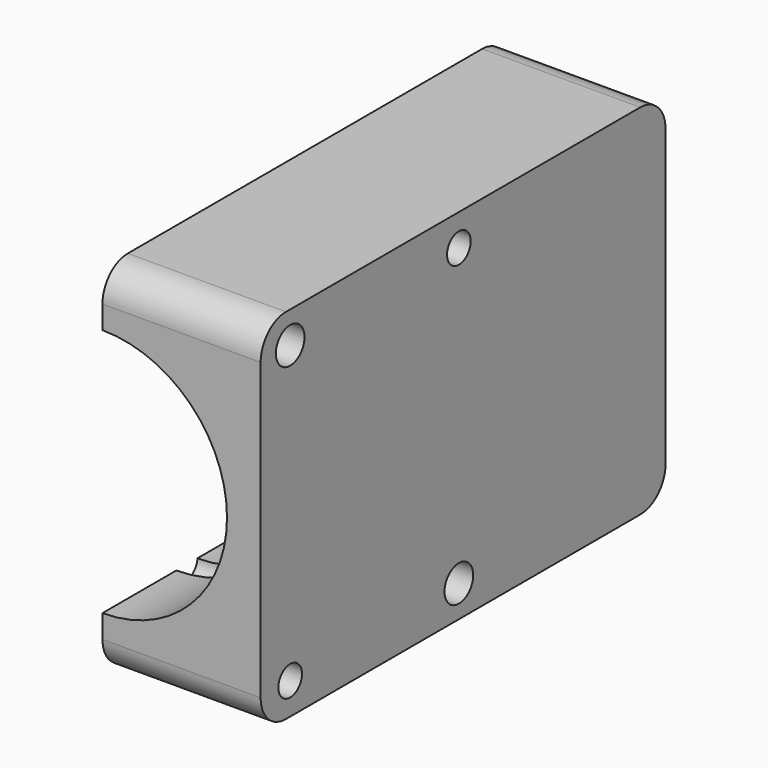
from build123d import *

# Parameters (mm, degrees)
F1_DEPTH      = 10
F1_DEPTH_BACK = 10
F5_DEPTH      = 28
F8_D          = 2.8
F8_ON_F2_D    = 2.8
F9_D          = 3.4
F9_ON_F2_D    = 3.4
F10_DEPTH     = 10
F11_F1_R      = 3
F11_F2_R      = 3
F11_F3_R      = 3
F11_F4_R      = 3
F11_F5_R      = 3
F11_F6_R      = 3
F12_DEPTH     = 10


with BuildPart() as f1:
    # F0 (on Front) → F1 (new body, two sides)
    with BuildSketch(Plane.XZ) as f1_sk:
        with BuildLine():
            Line((15, 17), (0, 17))
            Line((0, 17), (0, 11.81))
            ThreePointArc((0, 11.81), (8.3509310858, 8.3509310858), (11.81, 0))
            ThreePointArc((11.81, 0), (8.3509310858, -8.3509310858), (0, -11.81))
            Line((0, -11.81), (0, -17))
            Line((0, -17), (15, -17))
            Line((15, -17), (15, 17))
        make_face()
    extrude(amount=F1_DEPTH)
    extrude(f1_sk.sketch, amount=-F1_DEPTH_BACK)

    # F2 (on face) → F3 (revolve, cut)
    with BuildSketch(Plane(origin=(0, 0, 0), x_dir=(0, -1, 0), z_dir=(-1, 0, 0))):
        with BuildLine():
            Line((-1.25, -11.81), (1.25, -11.81))
            ThreePointArc((1.25, -11.81), (0, -10.56), (-1.25, -11.81))
        make_face()
        with BuildLine():
            ThreePointArc((-1.25, -11.81), (0, -13.06), (1.25, -11.81))
            Line((1.25, -11.81), (-1.25, -11.81))
        make_face()
    revolve(axis=Axis((0, 0, 0), (0, -1, 0)), mode=Mode.SUBTRACT)

    # F4 (on face) → F5 (join)
    with BuildSketch(Plane(origin=(0, 10, 0), x_dir=(-1, 0, 0), z_dir=(0, 1, 0))):
        with BuildLine():
            Line((0, -11.81), (0, 11.81))
            ThreePointArc((0, 11.81), (-11.81, 0), (0, -11.81))
        make_face()
        with BuildLine():
            Line((0, 17), (-15, 17))
            Line((-15, 17), (-15, -17))
            Line((-15, -17), (0, -17))
            Line((0, -17), (0, -11.81))
            ThreePointArc((0, -11.81), (-11.81, 0), (0, 11.81))
            Line((0, 11.81), (0, 17))
        make_face()
    extrude(amount=F5_DEPTH)

    # F6: union 

    # F8 (through all)
    with Locations(Plane(origin=(0, 0, 0), x_dir=(0, -1, 0), z_dir=(-1, 0, 0))):
        with Locations((-13.5, 14)):
            Hole(F8_D / 2)

    # F8 on F2 (through all)
    with Locations(Plane(origin=(0, 0, 0), x_dir=(0, -1, 0), z_dir=(-1, 0, 0))):
        with Locations((6.5, -14)):
            Hole(F8_ON_F2_D / 2)

    # F9 (through all)
    with Locations(Plane(origin=(0, 0, 0), x_dir=(0, -1, 0), z_dir=(-1, 0, 0))):
        with Locations((-13.5, -14)):
            Hole(F9_D / 2)

    # F9 on F2 (through all)
    with Locations(Plane(origin=(0, 0, 0), x_dir=(0, -1, 0), z_dir=(-1, 0, 0))):
        with Locations((6.5, 14)):
            Hole(F9_ON_F2_D / 2)

    # F7 (on face) → F10 (cut)
    with BuildSketch(Plane(origin=(0, 0, 0), x_dir=(0, -1, 0), z_dir=(-1, 0, 0))):
        with BuildLine():
            Line((-38, 11.75), (-38, -11.75))
            Line((-38, -11.75), (-25.1889491158, -11.75))
            ThreePointArc((-25.1889491158, -11.75), (-35.81, 0), (-25.1889491158, 11.75))
            Line((-25.1889491158, 11.75), (-38, 11.75))
        make_face()
        with BuildLine():
            ThreePointArc((-25.1889491158, 11.75), (-35.81, 0), (-25.1889491158, -11.75))
            Line((-25.1889491158, -11.75), (-24, -11.75))
            Line((-24, -11.75), (-24, 11.75))
            Line((-24, 11.75), (-25.1889491158, 11.75))
        make_face()
    extrude(amount=-F10_DEPTH, mode=Mode.SUBTRACT)

    # F11: fillet of radius 3 on 6 edges, made by hand

    # F11_f1
    f11_f1_edges = [f1.edges().sort_by_distance(p)[0] for p in [
        (5, 38, 11.75),
    ]]
    fillet(f11_f1_edges, radius=F11_F1_R)

    # F11_f2
    f11_f2_edges = [f1.edges().sort_by_distance(p)[0] for p in [
        (5, 38, -11.75),
    ]]
    fillet(f11_f2_edges, radius=F11_F2_R)

    # F11_f3
    f11_f3_edges = [f1.edges().sort_by_distance(p)[0] for p in [
        (7.5, -10, 17),
    ]]
    fillet(f11_f3_edges, radius=F11_F3_R)

    # F11_f4
    f11_f4_edges = [f1.edges().sort_by_distance(p)[0] for p in [
        (7.5, 38, 17),
    ]]
    fillet(f11_f4_edges, radius=F11_F4_R)

    # F11_f5
    f11_f5_edges = [f1.edges().sort_by_distance(p)[0] for p in [
        (7.5, -10, -17),
    ]]
    fillet(f11_f5_edges, radius=F11_F5_R)

    # F11_f6
    f11_f6_edges = [f1.edges().sort_by_distance(p)[0] for p in [
        (7.5, 38, -17),
    ]]
    fillet(f11_f6_edges, radius=F11_F6_R)

    # F7 (on face) → F12 (cut)
    with BuildSketch(Plane(origin=(0, 0, 0), x_dir=(0, -1, 0), z_dir=(-1, 0, 0))):
        with BuildLine():
            Line((-24, -11.75), (-25.1889491158, -11.75))
            ThreePointArc((-25.1889491158, -11.75), (-16.0805741704, -8.7612096499), (-12.19, 0))
            ThreePointArc((-12.19, 0), (-16.0805741704, 8.7612096499), (-25.1889491158, 11.75))
            Line((-25.1889491158, 11.75), (-24, 11.75))
            Line((-24, 11.75), (-24, -11.75))
        make_face()
    extrude(amount=-F12_DEPTH, mode=Mode.SUBTRACT)


solid = f1.part
